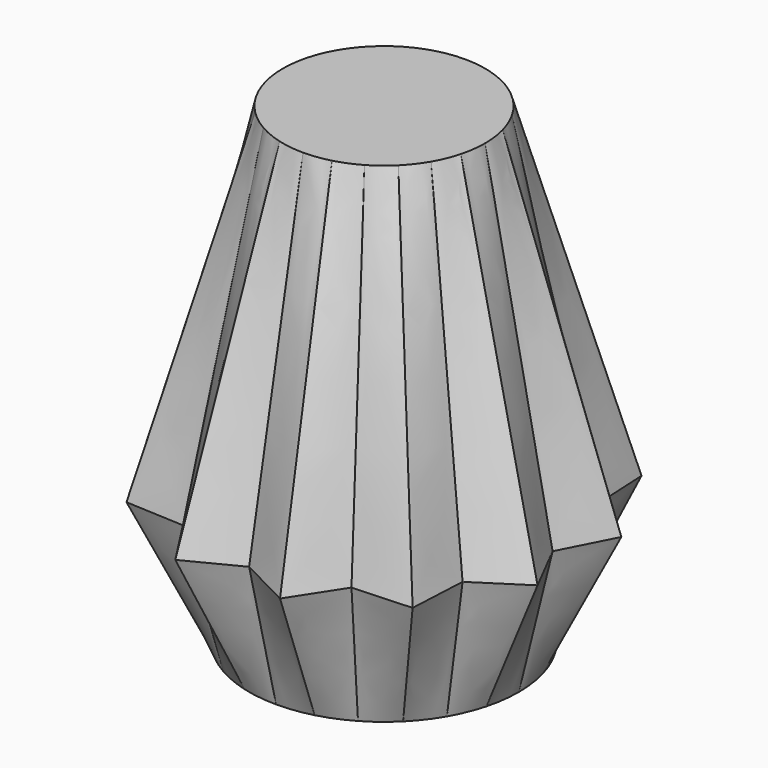
from build123d import *

# Parameters (mm, degrees)
F0_R = 20
F5_R = 15


# Not quite as in the source:
# - a feature of the source that left no trace in its solid (it failed there, or was rolled back) is left out


with BuildPart() as f3:
    # F2 (on offset) → F3 section 0
    with BuildSketch(Plane.XY.offset(20)):
        Polygon((12.5, 21.6506350946), (7.7645713531, 28.9777747887), (0, 25), (-7.7645713531, 28.9777747887), (-12.5, 21.6506350946), (-21.2132034356, 21.2132034356), (-21.6506350946, 12.5), (-28.9777747887, 7.7645713531), (-25, 0), (-28.9777747887, -7.7645713531), (-21.6506350946, -12.5), (-21.2132034356, -21.2132034356), (-12.5, -21.6506350946), (-7.7645713531, -28.9777747887), (0, -25), (7.7645713531, -28.9777747887), (12.5, -21.6506350946), (21.2132034356, -21.2132034356), (21.6506350946, -12.5), (28.9777747887, -7.7645713531), (25, 0), (28.9777747887, 7.7645713531), (21.6506350946, 12.5), (21.2132034356, 21.2132034356), align=None)
    # F0 (on Top) → F3 section 1
    with BuildSketch(Plane.XY):
        Circle(F0_R)
    loft()

    # F5 (on offset) → F6 section 0
    with BuildSketch(Plane.XY.offset(70)):
        Circle(F5_R)
    # F3_face (on face) → F6 section 1
    with BuildSketch(Plane.XY.offset(20)):
        Polygon((12.5, 21.6506350946), (7.7645713531, 28.9777747887), (0, 25), (-7.7645713531, 28.9777747887), (-12.5, 21.6506350946), (-21.2132034356, 21.2132034356), (-21.6506350946, 12.5), (-28.9777747887, 7.7645713531), (-25, 0), (-28.9777747887, -7.7645713531), (-21.6506350946, -12.5), (-21.2132034356, -21.2132034356), (-12.5, -21.6506350946), (-7.7645713531, -28.9777747887), (0, -25), (7.7645713531, -28.9777747887), (12.5, -21.6506350946), (21.2132034356, -21.2132034356), (21.6506350946, -12.5), (28.9777747887, -7.7645713531), (25, 0), (28.9777747887, 7.7645713531), (21.6506350946, 12.5), (21.2132034356, 21.2132034356), align=None)
    loft()


solid = f3.part
